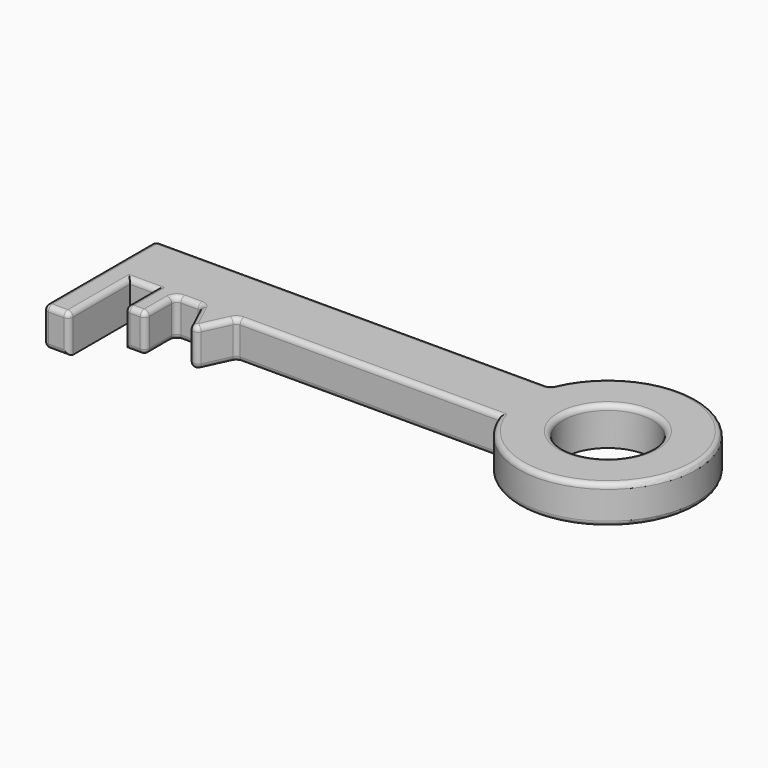
from build123d import *

# Parameters (mm, degrees)
F0_R     = 17.5
F0_W     = 10
F0_H     = 30
F0_W_2   = 8
F0_H_2   = 15
F1_DEPTH = 15
F2_R     = 2


with BuildPart() as f1:
    # F0 (on Top) → F1 (new body)
    with BuildSketch(Plane.XY):
        Polygon((64.8791989386, 52.4091998301), (-90.1208010614, 52.4091998301), (-90.1208010614, 27.4091998301), (-80.1208010614, 27.4091998301), (-70.1208010614, 27.4091998301), (-62.1208010614, 27.4091998301), (-52.1208010614, 27.4091998301), (-45.1209302745, 27.4091998301), (-38.1208010614, 27.4091998301), (64.8791989386, 27.4091998301), align=None)
        with BuildLine():
            ThreePointArc((64.8791989386, 27.4091998301), (132.5709410152, 39.9091998301), (64.8791989386, 52.4091998301))
            Line((64.8791989386, 52.4091998301), (64.8791989386, 27.4091998301))
        make_face()
        with Locations((97.5709410152, 39.9091998301)):
            Circle(F0_R, mode=Mode.SUBTRACT)
        with Locations((-85.1208010614, 12.4091998301)):
            Rectangle(F0_W, F0_H)
        Polygon((-45.1209302745, 12.4091998301), (-38.1208010614, 27.4091998301), (-45.1209302745, 27.4091998301), (-52.1208010614, 27.4091998301), align=None)
        with Locations((-66.1208010614, 19.9091998301)):
            Rectangle(F0_W_2, F0_H_2)
    extrude(amount=F1_DEPTH)

    # F2
    f2_edges = [f1.edges().sort_by_distance(p)[0] for p in [
        (-75.120801, 27.4092, 15),
        (-70.120801, 19.9092, 15),
        (-62.120801, 19.9092, 15),
        (-66.120801, 12.4092, 0),
        (-62.120801, 12.4092, 7.5),
        (-70.120801, 12.4092, 7.5),
        (-80.120801, 12.4092, 15),
        (-85.120801, -2.5908, 15),
        (-85.120801, -2.5908, 0),
        (-90.120801, -2.5908, 7.5),
        (-80.120801, -2.5908, 7.5),
        (-75.120801, 27.4092, 0),
        (-66.120801, 12.4092, 15),
        (-12.620801, 52.4092, 15),
        (-90.120801, 24.9092, 15),
        (-57.120801, 27.4092, 15),
        (-48.620866, 19.9092, 15),
        (-41.620866, 19.9092, 15),
        (13.379199, 27.4092, 15),
        (132.570941, 39.9092, 15),
        (80.070941, 39.9092, 15),
        (-45.12093, 12.4092, 7.5),
        (-38.120801, 27.4092, 7.5),
        (-41.620866, 19.9092, 0),
        (-48.620866, 19.9092, 0),
        (13.379199, 27.4092, 0),
        (132.570941, 39.9092, 0),
        (-12.620801, 52.4092, 0),
        (64.879199, 52.4092, 7.5),
        (-90.120801, 52.4092, 7.5),
        (-90.120801, 24.9092, 0),
        (-62.120801, 27.4092, 7.5),
        (-62.120801, 19.9092, 0),
        (-52.120801, 27.4092, 7.5),
        (-57.120801, 27.4092, 0),
    ]]
    fillet(f2_edges, radius=F2_R)


solid = f1.part
